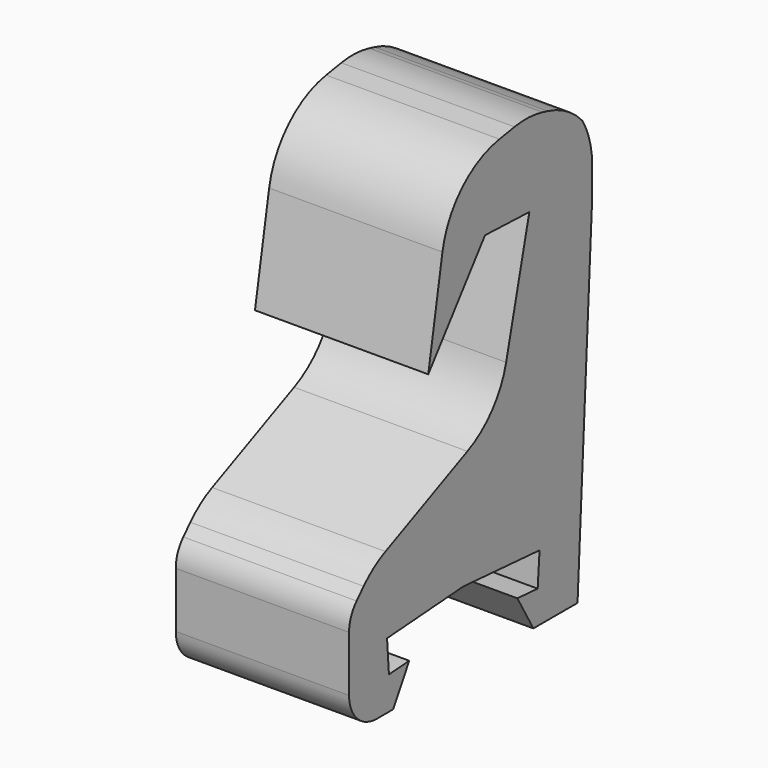
from build123d import *

# Parameters (mm, degrees)
F2_DEPTH     = 10
F3_T1_DEPTH  = 10
F3_T3_DEPTH  = 10.6551499426
F3_T5_DEPTH  = 18.2363272352
F3_T7_DEPTH  = 18.9745597366
F3_T9_DEPTH  = 15.1812109951
F3_T11_DEPTH = 27.7044164166
F3_T13_DEPTH = 14.9256552594
F4_R         = 2


# Not quite as in the source:
# - a fillet or chamfer that OpenCascade refuses, or shapes differently, is made with other operations: its cross-section is extruded or revolved along the edge and cut away or added


with BuildPart() as f2:
    # F1 (on Right) → F2 (new body)
    with BuildSketch(Plane.YZ):
        Polygon((-5.0547005384, 0), (-3.9, 2), (-5.3636236598, 1.894673786), (-5.5, 3.7897731222), (0, 4.18556761), (5.5, 3.7897731222), (5.3636236598, 1.894673786), (3.9, 2), (5.0547005384, 0), (8.2396483049, 0), (9.3, 20.2171942833), (9.3, 23.4340857714), (7.8309578478, 25.4216119647), (4.720045685, 26.1993408203), (-0.8888025768, 25.2726981416), (-2.5269729085, 15.9901147708), (1.5650866553, 21.3901147708), (4.7629482978, 21.2731493252), (2.5189220905, 11.9409952313), (-6.5113636665, 7.8363195062), (-8.2396483049, 6), (-8.2396483049, 0), align=None)
    extrude(amount=F2_DEPTH)

    # F3: fillet of radius 5 on 7 edges, made by hand

    # F3_s2 → F3_t1 (join)
    with BuildSketch(Plane.YZ):
        with BuildLine():
            ThreePointArc((3.0895210417, 14.313925334), (2.0840852214, 12.299936757), (0.2971092897, 10.9310802281))
            Line((0.2971092897, 10.9310802281), (2.5189220905, 11.9409952313))
            Line((2.5189220905, 11.9409952313), (3.0895210417, 14.313925334))
        make_face()
    extrude(amount=F3_T1_DEPTH)

    # F3_s4 → F3_t3 (cut)
    with BuildSketch(Plane.YZ.offset(-0.3275749713)):
        with BuildLine():
            ThreePointArc((9.2931371699, 20.0863441421), (9.298283998, 20.2172392528), (9.3, 20.3482242718))
            Line((9.3, 20.3482242718), (9.3, 20.2171942833))
            Line((9.3, 20.2171942833), (9.2931371699, 20.0863441421))
        make_face()
    extrude(amount=F3_T3_DEPTH, mode=Mode.SUBTRACT)

    # F3_s6 → F3_t5 (cut)
    with BuildSketch(Plane.YZ.offset(-4.1181636176)):
        with BuildLine():
            ThreePointArc((9.3, 21.7868203244), (9.0489155839, 23.3513652349), (8.3208796893, 24.7587770072))
            Line((8.3208796893, 24.7587770072), (9.3, 23.4340857714))
            Line((9.3, 23.4340857714), (9.3, 21.7868203244))
        make_face()
    extrude(amount=F3_T5_DEPTH, mode=Mode.SUBTRACT)

    # F3_s8 → F3_t7 (cut)
    with BuildSketch(Plane.YZ.offset(-4.4872798683)):
        with BuildLine():
            ThreePointArc((6.089637591, 25.856942485), (7.6572398301, 25.1619533788), (8.8978379592, 23.9781869661))
            Line((8.8978379592, 23.9781869661), (7.8309578478, 25.4216119647))
            Line((7.8309578478, 25.4216119647), (6.089637591, 25.856942485))
        make_face()
    extrude(amount=F3_T7_DEPTH, mode=Mode.SUBTRACT)

    # F3_s10 → F3_t9 (cut)
    with BuildSketch(Plane.YZ.offset(-2.5906054975)):
        with BuildLine():
            ThreePointArc((3.6976623422, 26.0304319828), (4.715730589, 26.0931776147), (5.7253482208, 25.948014923))
            Line((5.7253482208, 25.948014923), (4.720045685, 26.1993408203))
            Line((4.720045685, 26.1993408203), (3.6976623422, 26.0304319828))
        make_face()
    extrude(amount=F3_T9_DEPTH, mode=Mode.SUBTRACT)

    # F3_s12 → F3_t11 (cut)
    with BuildSketch(Plane.YZ.offset(-8.8522082083)):
        with BuildLine():
            ThreePointArc((-1.5041807088, 21.7856988327), (-0.0963977073, 24.4715707073), (2.6047244105, 25.8498667607))
            Line((2.6047244105, 25.8498667607), (-0.8888025768, 25.2726981416))
            Line((-0.8888025768, 25.2726981416), (-1.5041807088, 21.7856988327))
        make_face()
    extrude(amount=F3_T11_DEPTH, mode=Mode.SUBTRACT)

    # F3_s14 → F3_t13 (cut)
    with BuildSketch(Plane.YZ.offset(-2.4628276297)):
        with BuildLine():
            ThreePointArc((-5.6145333952, 8.2439696673), (-6.4554211776, 7.7581509396), (-7.1865343837, 7.1189439476))
            Line((-7.1865343837, 7.1189439476), (-6.5113636665, 7.8363195062))
            Line((-6.5113636665, 7.8363195062), (-5.6145333952, 8.2439696673))
        make_face()
    extrude(amount=F3_T13_DEPTH, mode=Mode.SUBTRACT)

    # F4
    f4_edges = [f2.edges().sort_by_distance(p)[0] for p in [
        (5, -8.239648, 0),
        (5, -8.239648, 6),
    ]]
    fillet(f4_edges, radius=F4_R)


solid = f2.part
